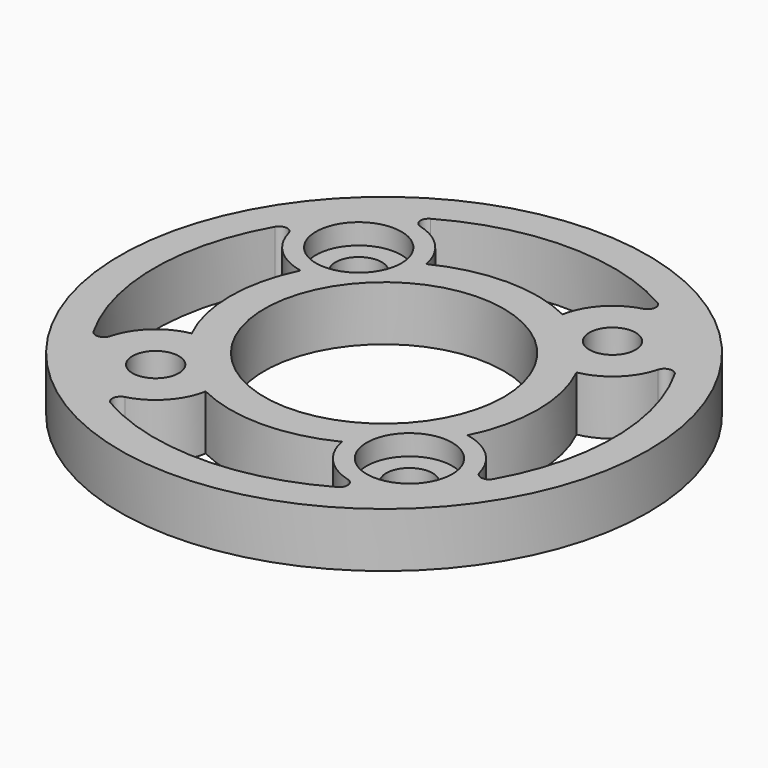
from build123d import *

# Parameters (mm, degrees)
F0_R            = 24.51608
F0_R_2          = 2.15265
F0_R_3          = 11.1125
F1_DEPTH        = 5.08
F3_DEPTH        = 5.08
F3_COPIES_COUNT = 4
F4_R            = 0.762
F6_R            = 3.96875
F7_DEPTH        = 1.905


# Not quite as in the source:
# - a pattern or mirror of a feature is missing from the dataset's text; its kind, count and spacing are read off the source's solid


with BuildPart() as f1:
    # F0 (on Top) → F1 (new body)
    with BuildSketch(Plane.XY):
        Circle(F0_R)
        with Locations((-11.7865906, -11.7865906)):
            Circle(F0_R_2, mode=Mode.SUBTRACT)
        with Locations((11.7865906, -11.7865906)):
            Circle(F0_R_2, mode=Mode.SUBTRACT)
        with Locations((-11.7865906, 11.7865906)):
            Circle(F0_R_2, mode=Mode.SUBTRACT)
        Circle(F0_R_3, mode=Mode.SUBTRACT)
        with Locations((11.7865906, 11.7865906)):
            Circle(F0_R_2, mode=Mode.SUBTRACT)
    extrude(amount=F1_DEPTH)

    # F2 (on face) → F3 (cut, through all)
    with BuildSketch(Plane.XY.offset(5.08)):
        with BuildLine():
            ThreePointArc((-12.5005198818, 17.2967828873), (-8.5209455851, 16.2818633057), (-6.3255779254, 12.810921909))
            ThreePointArc((-6.3255779254, 12.810921909), (0, 14.2875), (6.3255779254, 12.810921909))
            ThreePointArc((6.3255779254, 12.810921909), (8.5209455851, 16.2818633057), (12.5005198818, 17.2967828873))
            ThreePointArc((12.5005198818, 17.2967828873), (0, 21.34108), (-12.5005198818, 17.2967828873))
        make_face()
    f3 = extrude(amount=-F3_DEPTH, mode=Mode.SUBTRACT)

    # F3_copies: F3 ×4 about axis
    f3_copies_axis = Axis((0, 0, 0), (0, 0, 1))
    for i in range(1, F3_COPIES_COUNT):
        add(f3.rotate(f3_copies_axis, i * 360 / F3_COPIES_COUNT), mode=Mode.SUBTRACT)

    # F4
    f4_edges = [f1.edges().sort_by_distance(p)[0] for p in [
        (-12.50052, 17.296783, 2.54),
        (12.50052, 17.296783, 2.54),
        (-17.296783, 12.50052, 2.54),
        (-17.296783, -12.50052, 2.54),
        (-12.50052, -17.296783, 2.54),
        (12.50052, -17.296783, 2.54),
        (17.296783, -12.50052, 2.54),
        (17.296783, 12.50052, 2.54),
    ]]
    fillet(f4_edges, radius=F4_R)

    # F6 (on face) → F7 (cut, through all)
    with BuildSketch(Plane.XY.offset(5.08)):
        with Locations((11.7865906, -11.7865906)):
            Circle(F6_R)
        with Locations((-11.7865906, 11.7865906)):
            Circle(F6_R)
    extrude(amount=-F7_DEPTH, mode=Mode.SUBTRACT)


solid = f1.part
